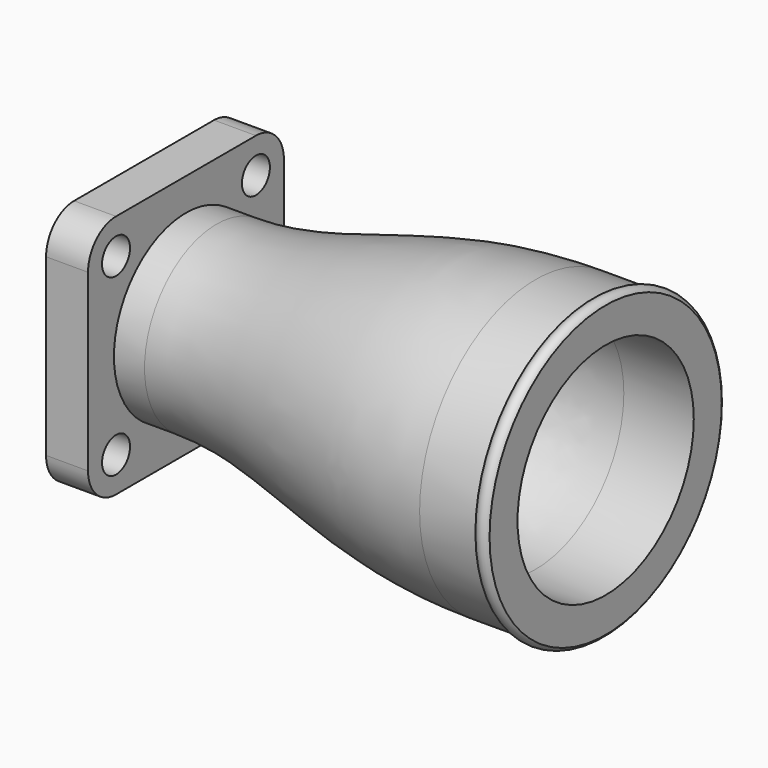
from build123d import *

# Parameters (mm, degrees)
F0_R     = 3.175
F0_R_2   = 10
F1_DEPTH = 7.62
F4_DEPTH = 12.7


with BuildPart() as f1:
    # F0 (on Right) → F1 (new body)
    with BuildSketch(Plane.YZ):
        with BuildLine():
            Line((-15.875, -22.225), (15.875, -22.225))
            ThreePointArc((15.875, -22.225), (20.3651280605, -20.3651280605), (22.225, -15.875))
            Line((22.225, -15.875), (22.225, 15.875))
            ThreePointArc((22.225, 15.875), (20.3651280605, 20.3651280605), (15.875, 22.225))
            Line((15.875, 22.225), (-15.875, 22.225))
            ThreePointArc((-15.875, 22.225), (-20.3651280605, 20.3651280605), (-22.225, 15.875))
            Line((-22.225, 15.875), (-22.225, -15.875))
            ThreePointArc((-22.225, -15.875), (-20.3651280605, -20.3651280605), (-15.875, -22.225))
        make_face()
        with Locations((-15.875, -15.875)):
            Circle(F0_R, mode=Mode.SUBTRACT)
        with Locations((15.875, -15.875)):
            Circle(F0_R, mode=Mode.SUBTRACT)
        with Locations((-15.875, 15.875)):
            Circle(F0_R, mode=Mode.SUBTRACT)
        Circle(F0_R_2, mode=Mode.SUBTRACT)
        with Locations((15.875, 15.875)):
            Circle(F0_R, mode=Mode.SUBTRACT)
    extrude(amount=-F1_DEPTH)

    # F2 (on Top) → F3 (revolve)
    with BuildSketch(Plane.XY):
        with BuildLine():
            Line((0, 16.35), (0, 15.875))
            Line((0, 15.875), (0, 10))
            Line((0, 10), (5.55625, 10))
            add(Edge.make_bspline(
                [(5.55625, 10), (25.4, 10), (38.1, 20), (63.5, 20)],
                knots=[0, 0, 0, 0, 58.8003245234, 58.8003245234, 58.8003245234, 58.8003245234], degree=3))
            Line((63.5, 20), (63.5, 26.35))
            add(Edge.make_bspline(
                [(5.55625, 16.35), (7.7700520833, 16.35), (11.9934239058, 16.6272658608), (18.0716052534, 17.6903425028), (24.2003826751, 19.2417667266), (30.6290469176, 21.0975445604), (37.5720151418, 23.0272233291), (45.2211301026, 24.7617582311), (53.7463141195, 26.0162490362), (60.1166666667, 26.35), (63.5, 26.35)],
                knots=[0, 0, 0, 0, 0.125, 0.25, 0.375, 0.5, 0.625, 0.75, 0.875, 1, 1, 1, 1], degree=3))
            Line((5.55625, 16.35), (0, 16.35))
        make_face()
    revolve(axis=Axis((31.75, 0, 0), (1, 0, 0)))

    # F4 (add): a face of the model
    f4_faces = [f1.faces().sort_by_distance(p)[0] for p in [
        (63.5, -20.7452905474, 0),
    ]]
    extrude(f4_faces, amount=F4_DEPTH)

    # F5 (on Top) → F6 (revolve)
    with BuildSketch(Plane.XY):
        with BuildLine():
            Line((73.66, 26.35), (76.2, 26.35))
            ThreePointArc((76.2, 26.35), (74.93, 27.112), (73.66, 26.35))
        make_face()
    revolve(axis=Axis((38.1, 0, 0), (1, 0, 0)))


solid = f1.part
